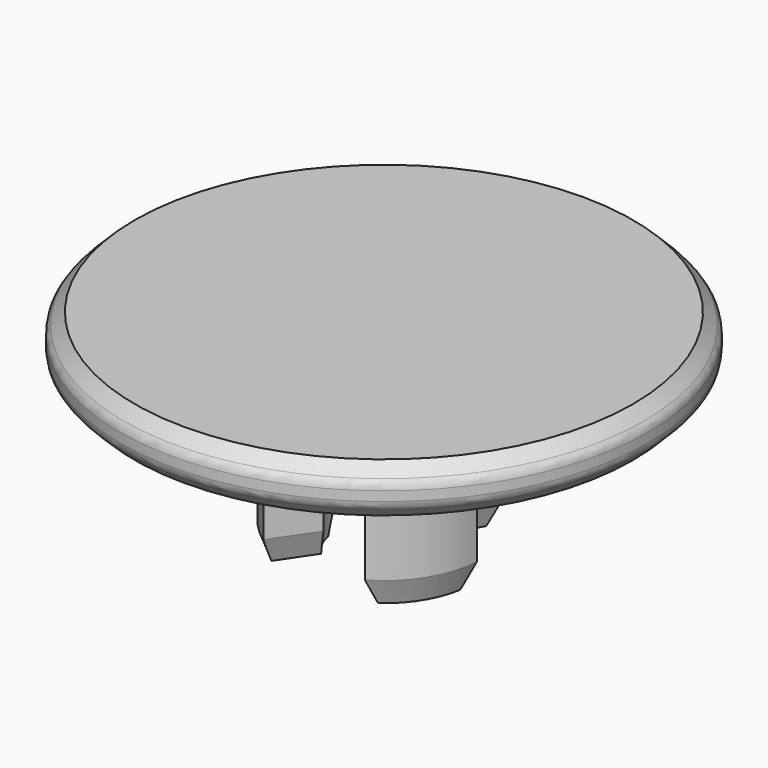
from build123d import *

# Parameters (mm, degrees)
F3_DEPTH    = 5
F4_C1_SIZE2 = 0.3639702343
F4_C1_SIZE  = 1
F4_C2_SIZE2 = 0.3639702343
F4_C2_SIZE  = 1
F4_C3_SIZE2 = 0.3639702343
F4_C3_SIZE  = 1
F4_C4_SIZE2 = 0.3639702343
F4_C4_SIZE  = 1
F4_C5_SIZE2 = 0.3639702343
F4_C5_SIZE  = 1
F4_C6_SIZE2 = 1
F4_C6_SIZE  = 0.3639702343
F4_C7_SIZE2 = 0.3639702343
F4_C7_SIZE  = 1
F4_C8_SIZE2 = 1
F4_C8_SIZE  = 0.3639702343
F4_C9_SIZE2 = 0.3639702343
F4_C9_SIZE  = 1
F5_SIZE     = 0.6
F6_R        = 0.5


with BuildPart() as f1:
    # F0 (on Front) → F1 (revolve)
    with BuildSketch(Plane.XZ):
        Polygon((10.7, 8.5), (0, 8.5), (0, 5), (2, 5), (2, 0), (4, 0), (4, 6), (6, 6), (6, 6.5), (10.7, 6.5), align=None)
    revolve(axis=Axis((0, 0, 6.75), (0, 0, -1)))

    # F2 (on face) → F3 (cut)
    with BuildSketch(Plane(origin=(0, 0, 0), x_dir=(1, 0, 0), z_dir=(0, 0, -1))):
        with BuildLine():
            ThreePointArc((4, 0), (3.4641016151, -2), (2, -3.4641016151))
            Line((2, -3.4641016151), (3, -5.1961524227))
            Line((3, -5.1961524227), (5.9853843016, 0.4185388425))
            Line((5.9853843016, 0.4185388425), (3.990256201, 0.279025895))
            ThreePointArc((3.990256201, 0.279025895), (3.9975633081, 0.1395979868), (4, 0))
        make_face()
        with BuildLine():
            ThreePointArc((-2.2367716139, 3.3161502902), (-0.1395979868, 3.9975633081), (2, 3.4641016151))
            Line((2, 3.4641016151), (3, 5.1961524227))
            Line((3, 5.1961524227), (-3.3551574208, 4.9742254353))
            Line((-3.3551574208, 4.9742254353), (-2.2367716139, 3.3161502902))
        make_face()
        with BuildLine():
            ThreePointArc((-0.8767422936, -1.7975880926), (-1.6960961923, -1.0598385285), (-2, 0))
            Line((-2, 0), (-4, 0))
            ThreePointArc((-4, 0), (-3.3921923846, -2.1196770569), (-1.7534845872, -3.5951761852))
            Line((-1.7534845872, -3.5951761852), (-0.8767422936, -1.7975880926))
        make_face()
        with BuildLine():
            ThreePointArc((-1.7534845872, -3.5951761852), (-3.3921923846, -2.1196770569), (-4, 0))
            Line((-4, 0), (-6, 0))
            Line((-6, 0), (-2.6302268807, -5.3927642778))
            Line((-2.6302268807, -5.3927642778), (-1.7534845872, -3.5951761852))
        make_face()
        with BuildLine():
            ThreePointArc((2, 0), (1.7320508076, -1), (1, -1.7320508076))
            Line((1, -1.7320508076), (2, -3.4641016151))
            ThreePointArc((2, -3.4641016151), (3.4641016151, -2), (4, 0))
            ThreePointArc((4, 0), (3.9975633081, 0.1395979868), (3.990256201, 0.279025895))
            Line((3.990256201, 0.279025895), (1.9951281005, 0.1395129475))
            ThreePointArc((1.9951281005, 0.1395129475), (1.998781654, 0.0697989934), (2, 0))
        make_face()
        with BuildLine():
            ThreePointArc((-1.1183858069, 1.6580751451), (-0.0697989934, 1.998781654), (1, 1.7320508076))
            Line((1, 1.7320508076), (2, 3.4641016151))
            ThreePointArc((2, 3.4641016151), (-0.1395979868, 3.9975633081), (-2.2367716139, 3.3161502902))
            Line((-2.2367716139, 3.3161502902), (-1.1183858069, 1.6580751451))
        make_face()
        with BuildLine():
            ThreePointArc((-0.4983586629, -1.0217866811), (-0.9640965616, -0.6024343936), (-1.1368418442, 0))
            Line((-1.1368418442, 0), (-2, 0))
            ThreePointArc((-2, 0), (-1.6960961923, -1.0598385285), (-0.8767422936, -1.7975880926))
            Line((-0.8767422936, -1.7975880926), (-0.4983586629, -1.0217866811))
        make_face()
        with BuildLine():
            Line((-0.4983586629, -1.0217866811), (0, 0))
            Line((0, 0), (-1.1368418442, 0))
            ThreePointArc((-1.1368418442, 0), (-0.9640965616, -0.6024343936), (-0.4983586629, -1.0217866811))
        make_face()
        with BuildLine():
            Line((-0.6357138916, 0.9424846029), (0, 0))
            Line((0, 0), (0.5684209221, 0.9845339171))
            ThreePointArc((0.5684209221, 0.9845339171), (-0.0396752082, 1.1361493108), (-0.6357138916, 0.9424846029))
        make_face()
        with BuildLine():
            ThreePointArc((-0.6357138916, 0.9424846029), (-0.0396752082, 1.1361493108), (0.5684209221, 0.9845339171))
            Line((0.5684209221, 0.9845339171), (1, 1.7320508076))
            ThreePointArc((1, 1.7320508076), (-0.0697989934, 1.998781654), (-1.1183858069, 1.6580751451))
            Line((-1.1183858069, 1.6580751451), (-0.6357138916, 0.9424846029))
        make_face()
        with BuildLine():
            Line((1.1340725546, 0.0793020783), (0, 0))
            Line((0, 0), (0.5684209221, -0.9845339171))
            ThreePointArc((0.5684209221, -0.9845339171), (0.9845339171, -0.5684209221), (1.1368418442, 0))
            ThreePointArc((1.1368418442, 0), (1.1361493108, 0.0396752082), (1.1340725546, 0.0793020783))
        make_face()
        with BuildLine():
            ThreePointArc((1.1368418442, 0), (0.9845339171, -0.5684209221), (0.5684209221, -0.9845339171))
            Line((0.5684209221, -0.9845339171), (1, -1.7320508076))
            ThreePointArc((1, -1.7320508076), (1.7320508076, -1), (2, 0))
            ThreePointArc((2, 0), (1.998781654, 0.0697989934), (1.9951281005, 0.1395129475))
            Line((1.9951281005, 0.1395129475), (1.1340725546, 0.0793020783))
            ThreePointArc((1.1340725546, 0.0793020783), (1.1361493108, 0.0396752082), (1.1368418442, 0))
        make_face()
    extrude(amount=-F3_DEPTH, mode=Mode.SUBTRACT)

    # F4: chamfer of 1 x 0.3639702343 on 9 edges, made by hand

    # F4_c1
    f4_c1_edges = [f1.edges().sort_by_distance(p)[0] for p in [
        (0.1395979868, 3.9975633081, 0),
    ]]
    f4_c1_side = f1.faces().sort_by_distance((0.1395979868, 3.9975633081, 0.0072794047))[0]
    chamfer(f4_c1_edges, length=F4_C1_SIZE, length2=F4_C1_SIZE2, reference=f4_c1_side)

    # F4_c2
    f4_c2_edges = [f1.edges().sort_by_distance(p)[0] for p in [
        (-3.5317903714, -1.8778862511, 0),
    ]]
    f4_c2_side = f1.faces().sort_by_distance((-3.5317903714, -1.8778862511, 0.0072794047))[0]
    chamfer(f4_c2_edges, length=F4_C2_SIZE, length2=F4_C2_SIZE2, reference=f4_c2_side)

    # F4_c3
    f4_c3_edges = [f1.edges().sort_by_distance(p)[0] for p in [
        (3.3921923846, -2.1196770569, 0),
    ]]
    f4_c3_side = f1.faces().sort_by_distance((3.3921923846, -2.1196770569, 0.0072794047))[0]
    chamfer(f4_c3_edges, length=F4_C3_SIZE, length2=F4_C3_SIZE2, reference=f4_c3_side)

    # F4_c4
    f4_c4_edges = [f1.edges().sort_by_distance(p)[0] for p in [
        (2.8111503402, -0.1965747812, 0),
    ]]
    f4_c4_side = f1.faces().sort_by_distance((2.8111503402, -0.1965747812, 0.0072794047))[0]
    chamfer(f4_c4_edges, length=F4_C4_SIZE, length2=F4_C4_SIZE2, reference=f4_c4_side)

    # F4_c5
    f4_c5_edges = [f1.edges().sort_by_distance(p)[0] for p in [
        (1.4090074414, 2.4404724768, 0),
    ]]
    f4_c5_side = f1.faces().sort_by_distance((1.4090074414, 2.4404724768, 0.0072794047))[0]
    chamfer(f4_c5_edges, length=F4_C5_SIZE, length2=F4_C5_SIZE2, reference=f4_c5_side)

    # F4_c6
    f4_c6_edges = [f1.edges().sort_by_distance(p)[0] for p in [
        (-1.2353364159, 2.5328149991, 0),
    ]]
    f4_c6_side = f1.faces().sort_by_distance((-1.2287937303, 2.5360060801, 0))[0]
    chamfer(f4_c6_edges, length=F4_C6_SIZE, length2=F4_C6_SIZE2, reference=f4_c6_side)

    # F4_c7
    f4_c7_edges = [f1.edges().sort_by_distance(p)[0] for p in [
        (-2.8180148829, 0, 0),
    ]]
    f4_c7_side = f1.faces().sort_by_distance((-2.8180148829, 0, 0.0072794047))[0]
    chamfer(f4_c7_edges, length=F4_C7_SIZE, length2=F4_C7_SIZE2, reference=f4_c7_side)

    # F4_c8
    f4_c8_edges = [f1.edges().sort_by_distance(p)[0] for p in [
        (-1.5758139244, -2.3362402179, 0),
    ]]
    f4_c8_side = f1.faces().sort_by_distance((-1.5818488244, -2.3321696265, 0))[0]
    chamfer(f4_c8_edges, length=F4_C8_SIZE, length2=F4_C8_SIZE2, reference=f4_c8_side)

    # F4_c9
    f4_c9_edges = [f1.edges().sort_by_distance(p)[0] for p in [
        (1.4090074414, -2.4404724768, 0),
    ]]
    f4_c9_side = f1.faces().sort_by_distance((1.4090074414, -2.4404724768, 0.0072794047))[0]
    chamfer(f4_c9_edges, length=F4_C9_SIZE, length2=F4_C9_SIZE2, reference=f4_c9_side)

    # F5
    f5_edges = [f1.edges().sort_by_distance(p)[0] for p in [
        (-10.7, 0, 8.5),
        (-10.7, 0, 6.5),
    ]]
    chamfer(f5_edges, length=F5_SIZE)

    # F6
    f6_edges = [f1.edges().sort_by_distance(p)[0] for p in [
        (10.7, 0, 7.5),
        (-10.7, 0, 7.1),
        (-10.7, 0, 7.9),
    ]]
    fillet(f6_edges, radius=F6_R)


solid = f1.part
